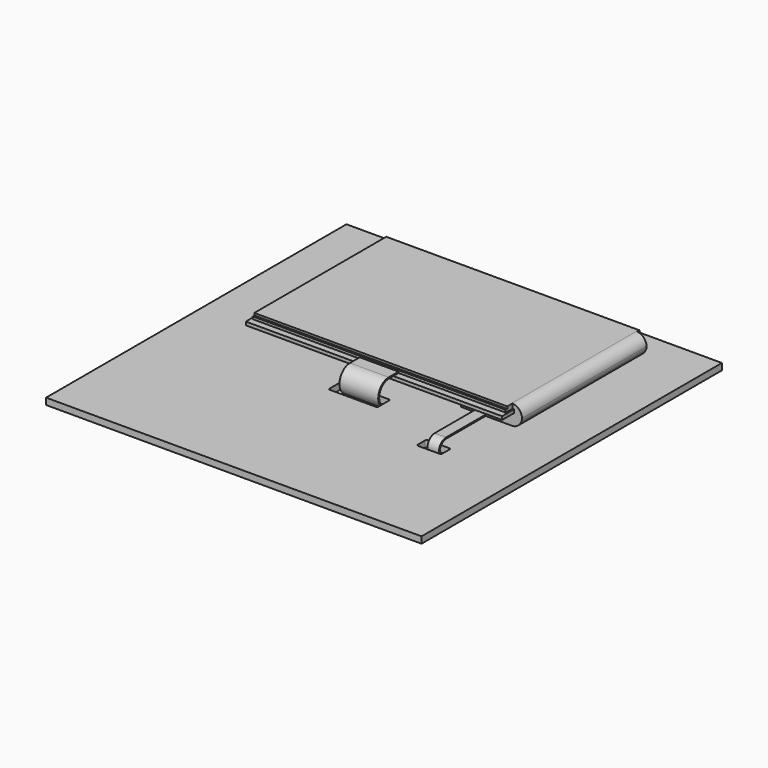
from build123d import *

# Parameters (mm, degrees)
F0_W         = 62.8
F0_H         = 42.82
F1_DEPTH     = 0.81
F2_W         = 15
F2_H         = 38.15
F3_DEPTH     = 2.9
F4_W         = 62
F4_H         = 41.22
F5_DEPTH     = 0.6
F6_W         = 62
F6_H         = 40.42
F7_DEPTH     = 0.54
F8_W         = 2.35
F8_H         = 38.15
F8_W_2       = 62
F9_DEPTH     = 1.95
F10_T1_DEPTH = 50.65
F13_W        = 92
F13_H        = 92
F14_DEPTH    = 1.6
F16_W        = 3
F16_H        = 2.9
F17_DEPTH    = 0.79
F11_W        = 2.8
F11_H        = 0.3
F22_DEPTH    = 1.6
F24_W        = 5.6
F24_H        = 3.4
F25_DEPTH    = 0.55
F23_W        = 9.5
F23_H        = 0.3
F30_DEPTH    = 1.6


# Not quite as in the source:
# - a fillet or chamfer that OpenCascade refuses, or shapes differently, is made with other operations: its cross-section is extruded or revolved along the edge and cut away or added


with BuildPart() as f1:
    # F0 (on Top) → F1 (new body)
    with BuildSketch(Plane.XY):
        Rectangle(F0_W, F0_H)
    extrude(amount=F1_DEPTH)

    # F2 (on face) → F3 (join)
    with BuildSketch(Plane(origin=(0, 0, 0), x_dir=(1, 0, 0), z_dir=(0, 0, -1))):
        with Locations((25.85, -1.335)):
            Rectangle(F2_W, F2_H)
    extrude(amount=F3_DEPTH)

    # F4 (on face) → F5 (join)
    with BuildSketch(Plane.XY.offset(0.81)):
        with Locations((0, 0.8)):
            Rectangle(F4_W, F4_H)
    extrude(amount=F5_DEPTH)

    # F6 (on face) → F7 (join)
    with BuildSketch(Plane.XY.offset(1.41)):
        with Locations((0, 0.9)):
            Rectangle(F6_W, F6_H)
    extrude(amount=F7_DEPTH)

    # F8 (on face) → F9 (join, through all)
    with BuildSketch(Plane.XY.offset(1.95)):
        with Locations((32.175, 1.335)):
            Rectangle(F8_W, F8_H)
        with Locations((0, 1.335)):
            Rectangle(F8_W_2, F8_H)
    extrude(amount=-F9_DEPTH)

    # F10: fillet of radius 2.5 on 2 edges, made by hand

    # F10_s2 → F10_t1 (cut)
    with BuildSketch(Plane.XZ.offset(-26.66)):
        with BuildLine():
            ThreePointArc((30.85, 1.95), (32.617766953, 1.217766953), (33.35, -0.55))
            Line((33.35, -0.55), (33.35, 1.95))
            Line((33.35, 1.95), (30.85, 1.95))
        make_face()
        with BuildLine():
            ThreePointArc((30.85, -2.9), (32.617766953, -2.167766953), (33.35, -0.4))
            Line((33.35, -0.4), (33.35, -2.9))
            Line((33.35, -2.9), (30.85, -2.9))
        make_face()
    extrude(amount=F10_T1_DEPTH, mode=Mode.SUBTRACT)

    # F20: sweep along a path in F19
    with BuildLine(Plane(origin=(24.7, 0, 0), x_dir=(0, -1, 0), z_dir=(-1, 0, 0))) as f20_path:
        Line((17.74, -1.35), (31.94, -1.35))
        ThreePointArc((31.94, -1.35), (33.985, -3.395), (31.94, -5.44))
        Line((31.94, -5.44), (19.3450039609, -5.44))
    # F11 (on face) → F20 (sweep)
    with BuildSketch(Plane.XZ.offset(17.74)):
        with Locations((24.7, -1.35)):
            Rectangle(F11_W, F11_H)
    sweep(path=f20_path.line)

    # F28: sweep along a path in F27
    with BuildLine(Plane.YZ) as f28_path:
        Line((-19.81, 0.96), (-21.41, 0.96))
        Line((-21.41, 0.96), (-22.81, 0.96))
        ThreePointArc((-22.81, 0.96), (-25.89, -2.12), (-22.81, -5.2))
        Line((-22.81, -5.2), (-19.41, -5.2))
    # F23 (on face) → F28 (sweep)
    with BuildSketch(Plane.XZ.offset(19.81)):
        with Locations((0, 0.96)):
            Rectangle(F23_W, F23_H)
    sweep(path=f28_path.line)


with BuildPart() as f14:
    # F13 (on face) → F14 (new body)
    with BuildSketch(Plane(origin=(0, 0, -2.9), x_dir=(1, 0, 0), z_dir=(0, 0, -1))):
        with Locations((0, 18.329)):
            Rectangle(F13_W, F13_H)
    extrude(amount=F14_DEPTH)

    # F16 (on face) → F17 (join)
    with BuildSketch(Plane(origin=(0, 0, -4.5), x_dir=(1, 0, 0), z_dir=(0, 0, -1))):
        with Locations((24.7, 20.7950039609)):
            Rectangle(F16_W, F16_H)
    extrude(amount=F17_DEPTH)

    # F21 (on face) → F22 (cut, through all)
    with BuildSketch(Plane.XY.offset(-2.9)):
        with BuildLine():
            ThreePointArc((27.7, -32.885), (27.5828427125, -32.6021572875), (27.3, -32.485))
            Line((27.3, -32.485), (22.1, -32.485))
            ThreePointArc((22.1, -32.485), (21.8171572875, -32.6021572875), (21.7, -32.885))
            Line((21.7, -32.885), (21.7, -35.085))
            ThreePointArc((21.7, -35.085), (21.8171572875, -35.3678427125), (22.1, -35.485))
            Line((22.1, -35.485), (27.3, -35.485))
            ThreePointArc((27.3, -35.485), (27.5828427125, -35.3678427125), (27.7, -35.085))
            Line((27.7, -35.085), (27.7, -32.885))
        make_face()
    extrude(amount=-F22_DEPTH, mode=Mode.SUBTRACT)

    # F24 (on face) → F25 (join)
    with BuildSketch(Plane(origin=(0, 0, -4.5), x_dir=(1, 0, 0), z_dir=(0, 0, -1))):
        with Locations((0, 21.11)):
            Rectangle(F24_W, F24_H)
    extrude(amount=F25_DEPTH)

    # F29 (on face) → F30 (cut, through all)
    with BuildSketch(Plane.XY.offset(-2.9)):
        with BuildLine():
            ThreePointArc((6, -24.29), (5.8828427125, -24.0071572875), (5.6, -23.89))
            Line((5.6, -23.89), (-5.6, -23.89))
            ThreePointArc((-5.6, -23.89), (-5.8828427125, -24.0071572875), (-6, -24.29))
            Line((-6, -24.29), (-6, -27.49))
            ThreePointArc((-6, -27.49), (-5.8828427125, -27.7728427125), (-5.6, -27.89))
            Line((-5.6, -27.89), (5.6, -27.89))
            ThreePointArc((5.6, -27.89), (5.8828427125, -27.7728427125), (6, -27.49))
            Line((6, -27.49), (6, -24.29))
        make_face()
    extrude(amount=-F30_DEPTH, mode=Mode.SUBTRACT)


solid = Compound([f1.part, f14.part])
